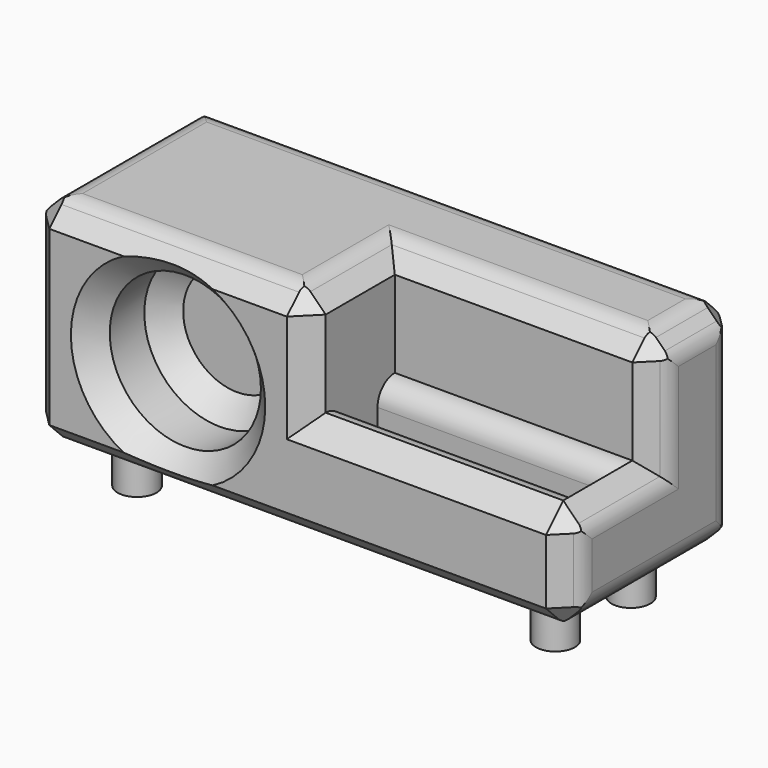
from build123d import *

# Parameters (mm, degrees)
F0_W         = 125
F0_H         = 50
F1_DEPTH     = 50
F2_W         = 60
F2_H         = 25
F3_DEPTH     = 25
F4_R         = 17.5
F5_DEPTH     = 20
F6_T3_DEPTH  = 6.3508529611
F6_T5_DEPTH  = 6.3508529611
F6_T7_DEPTH  = 6.3508529611
F6_T9_DEPTH  = 6.3508529611
F6_T11_DEPTH = 6.3508529611
F6_T13_DEPTH = 6.3508529611
F6_T15_DEPTH = 6.3508529611
F6_T17_DEPTH = 6.3508529611
F6_T19_DEPTH = 6.3508529611
F6_T21_DEPTH = 90.7168298797
F6_T23_DEPTH = 37.8584149398
F6_T25_DEPTH = 72.8584149398
F6_T27_DEPTH = 50.7168298797
F6_T29_DEPTH = 150.7168298797
F6_T31_DEPTH = 75.7168298797
F6_T33_DEPTH = 75.7168298797
F6_T35_DEPTH = 37.8584149398
F6_T37_DEPTH = 50.7168298797
F6_T45_DEPTH = 37.8584149398
F6_T49_DEPTH = 72.8584149398
F6_T56_DEPTH = 37.8584149398
F6_T60_DEPTH = 72.8584149398
F6_T67_DEPTH = 37.8584149398
F6_T71_DEPTH = 37.8584149398
F7_W         = 55
F7_H         = 10
F8_DEPTH     = 10
F9_T1_DEPTH  = 50.3553390594
F9_T3_DEPTH  = 125.3553390595
F9_T5_DEPTH  = 25.3553390594
F9_T7_DEPTH  = 65.3553390594
F9_T9_DEPTH  = 50.3553390593
F9_T11_DEPTH = 25.3553390595
F9_T16_DEPTH = 70.3553390595
F9_T21_DEPTH = 35.3553390594
F9_T26_DEPTH = 35.3553390594
F9_T31_DEPTH = 35.3553390595
F9_T37_DEPTH = 70.3553390595
F9_T41_DEPTH = 35.3553390594
F9_T48_DEPTH = 35.3553390594
F9_T52_DEPTH = 35.3553390595
F10_R        = 4.99999
F11_R        = 4.5
F12_DEPTH    = 10.1


# Not quite as in the source:
# - a fillet or chamfer that OpenCascade refuses, or shapes differently, is made with other operations: its cross-section is extruded or revolved along the edge and cut away or added
# - a fillet or chamfer is up to 0.001 mm smaller than in the source, because OpenCascade refuses the exact size


with BuildPart() as f1:
    # F0 (on Front) → F1 (new body)
    with BuildSketch(Plane.XZ):
        with Locations((4.2377149548, 2.7714315802)):
            Rectangle(F0_W, F0_H)
    extrude(amount=F1_DEPTH)

    # F2 (on face) → F3 (cut)
    with BuildSketch(Plane.XZ.offset(50)):
        with Locations((36.7377149548, 15.2714315802)):
            Rectangle(F2_W, F2_H)
    extrude(amount=-F3_DEPTH, mode=Mode.SUBTRACT)

    # F4 (on face) → F5 (cut)
    with BuildSketch(Plane.XZ.offset(50)):
        with Locations((-25.7622850452, 2.7714315802)):
            Circle(F4_R)
    extrude(amount=-F5_DEPTH, mode=Mode.SUBTRACT)

    # F6: chamfer of 5 on 20 edges, made by hand

    # F6_s1 → F6_t2 (revolve)
    with BuildSketch(Plane.XY.offset(2.7714315802)):
        Polygon((-8.2622850452, -35), (-13.2622850452, -30), (-8.2622850452, -30), align=None)
    revolve(axis=Axis((-25.7622850452, -30, 2.7714315802), (0, -1, 0)))

    # F6_s4 → F6_t3 (cut)
    with BuildSketch(Plane(origin=(24.8363821783, -24.8363821783, 24.8363821783), x_dir=(0.7071067812, 0.7071067812, 0), z_dir=(0.5773502692, -0.5773502692, 0.5773502692))):
        Polygon((-30.5910551251, 3.5946867022), (-34.126589031, -2.5290376548), (-27.0555212191, -2.5290376548), align=None)
    extrude(amount=F6_T3_DEPTH, mode=Mode.SUBTRACT)

    # F6_s6 → F6_t5 (cut)
    with BuildSketch(Plane(origin=(-42.0112388751, -42.0112388751, 42.0112388751), x_dir=(0.7071067812, -0.7071067812, 0), z_dir=(-0.5773502692, -0.5773502692, 0.5773502692))):
        Polygon((-5.8423177835, -17.4401309541), (-9.3778516895, -23.563855311), (-2.3067838776, -23.563855311), align=None)
    extrude(amount=F6_T5_DEPTH, mode=Mode.SUBTRACT)

    # F6_s8 → F6_t7 (cut)
    with BuildSketch(Plane(origin=(36.503048845, -36.503048845, 36.503048845), x_dir=(0.7071067812, 0.7071067812, 0), z_dir=(0.5773502692, -0.5773502692, 0.5773502692))):
        Polygon((29.5130212758, -10.694003464), (25.9774873699, -16.817727821), (33.0485551817, -16.817727821), align=None)
        Polygon((11.8353517461, -41.3126252488), (8.2998178402, -47.4363496058), (15.3708856521, -47.4363496058), align=None)
    extrude(amount=F6_T7_DEPTH, mode=Mode.SUBTRACT)

    # F6_s10 → F6_t9 (cut)
    with BuildSketch(Plane(origin=(28.1697155117, 28.1697155117, 28.1697155117), x_dir=(-0.7071067812, 0.7071067812, 0), z_dir=(0.5773502692, 0.5773502692, 0.5773502692))):
        Polygon((-47.1906908055, -0.4877962024), (-43.6551568995, -6.6115205594), (-50.7262247114, -6.6115205594), align=None)
    extrude(amount=F6_T9_DEPTH, mode=Mode.SUBTRACT)

    # F6_s12 → F6_t11 (cut)
    with BuildSketch(Plane(origin=(-25.3445722085, 25.3445722085, 25.3445722085), x_dir=(-0.7071067812, -0.7071067812, 0), z_dir=(-0.5773502692, 0.5773502692, 0.5773502692))):
        Polygon((41.1976568429, 2.9722835691), (37.6621229369, -3.1514407878), (44.7331907488, -3.1514407878), align=None)
    extrude(amount=F6_T11_DEPTH, mode=Mode.SUBTRACT)

    # F6_s14 → F6_t13 (cut)
    with BuildSketch(Plane(origin=(-40.1636178217, -40.1636178217, -40.1636178217), x_dir=(0.7071067812, -0.7071067812, 0), z_dir=(-0.5773502692, -0.5773502692, -0.5773502692))):
        Polygon((-9.3778516895, 28.08958413), (-2.3067838776, 28.08958413), (-5.8423177835, 21.9658597731), align=None)
    extrude(amount=F6_T13_DEPTH, mode=Mode.SUBTRACT)

    # F6_s16 → F6_t15 (cut)
    with BuildSketch(Plane(origin=(26.3220944582, 26.3220944582, -26.3220944582), x_dir=(-0.7071067812, 0.7071067812, 0), z_dir=(0.5773502692, 0.5773502692, -0.5773502692))):
        Polygon((-43.6551568995, 11.1372493784), (-50.7262247114, 11.1372493784), (-47.1906908055, 5.0135250214), align=None)
    extrude(amount=F6_T15_DEPTH, mode=Mode.SUBTRACT)

    # F6_s18 → F6_t17 (cut)
    with BuildSketch(Plane(origin=(42.9887611249, -42.9887611249, -42.9887611249), x_dir=(0.7071067812, 0.7071067812, 0), z_dir=(0.5773502692, -0.5773502692, -0.5773502692))):
        Polygon((8.2998178402, 31.5496639016), (15.3708856521, 31.5496639016), (11.8353517461, 25.4259395446), align=None)
    extrude(amount=F6_T17_DEPTH, mode=Mode.SUBTRACT)

    # F6_s20 → F6_t19 (cut)
    with BuildSketch(Plane(origin=(-23.496951155, 23.496951155, -23.496951155), x_dir=(-0.7071067812, -0.7071067812, 0), z_dir=(-0.5773502692, 0.5773502692, -0.5773502692))):
        Polygon((37.6621229369, 7.6771696068), (44.7331907488, 7.6771696068), (41.1976568429, 1.5534452499), align=None)
    extrude(amount=F6_T19_DEPTH, mode=Mode.SUBTRACT)

    # F6_s22 → F6_t21 (cut)
    with BuildSketch(Plane.YZ.offset(-71.120699985)):
        Polygon((-45, 27.7714315802), (-50, 22.7714315802), (-50, 27.7714315802), align=None)
    extrude(amount=F6_T21_DEPTH, mode=Mode.SUBTRACT)

    # F6_s24 → F6_t23 (cut)
    with BuildSketch(Plane.XZ.offset(25)):
        Polygon((1.7377149548, 27.7714315802), (6.7377149548, 22.7714315802), (6.7377149548, 27.7714315802), align=None)
        Polygon((66.7377149548, -2.2285684198), (61.7377149548, 2.7714315802), (66.7377149548, 2.7714315802), align=None)
    extrude(amount=F6_T23_DEPTH, mode=Mode.SUBTRACT)

    # F6_s26 → F6_t25 (cut)
    with BuildSketch(Plane.YZ.offset(6.7377149548)):
        Polygon((-20, 27.7714315802), (-25, 22.7714315802), (-25, 27.7714315802), align=None)
        Polygon((-50, -2.2285684198), (-45, 2.7714315802), (-50, 2.7714315802), align=None)
    extrude(amount=F6_T25_DEPTH, mode=Mode.SUBTRACT)

    # F6_s28 → F6_t27 (cut)
    with BuildSketch(Plane.XZ.offset(-12.8584149398)):
        Polygon((61.7377149548, 27.7714315802), (66.7377149548, 22.7714315802), (66.7377149548, 27.7714315802), align=None)
    extrude(amount=F6_T27_DEPTH, mode=Mode.SUBTRACT)

    # F6_s30 → F6_t29 (cut)
    with BuildSketch(Plane.YZ.offset(-71.120699985)):
        Polygon((-5, 27.7714315802), (0, 22.7714315802), (0, 27.7714315802), align=None)
        Polygon((-50, -17.2285684198), (-45, -22.2285684198), (-50, -22.2285684198), align=None)
        Polygon((0, -17.2285684198), (-5, -22.2285684198), (0, -22.2285684198), align=None)
    extrude(amount=F6_T29_DEPTH, mode=Mode.SUBTRACT)

    # F6_s32 → F6_t31 (cut)
    with BuildSketch(Plane.XZ.offset(-12.8584149398)):
        Polygon((-53.2622850452, 27.7714315802), (-58.2622850452, 22.7714315802), (-58.2622850452, 27.7714315802), align=None)
        Polygon((66.7377149548, -17.2285684198), (61.7377149548, -22.2285684198), (66.7377149548, -22.2285684198), align=None)
        Polygon((-58.2622850452, -17.2285684198), (-53.2622850452, -22.2285684198), (-58.2622850452, -22.2285684198), align=None)
    extrude(amount=F6_T31_DEPTH, mode=Mode.SUBTRACT)

    # F6_s34 → F6_t33 (cut)
    with BuildSketch(Plane.XY.offset(-35.0869833596)):
        Polygon((-58.2622850452, -45), (-53.2622850452, -50), (-58.2622850452, -50), align=None)
        Polygon((61.7377149548, 0), (66.7377149548, -5), (66.7377149548, 0), align=None)
        Polygon((-53.2622850452, 0), (-58.2622850452, -5), (-58.2622850452, 0), align=None)
    extrude(amount=F6_T33_DEPTH, mode=Mode.SUBTRACT)

    # F6_s36 → F6_t35 (cut)
    with BuildSketch(Plane.XY.offset(2.7714315802)):
        Polygon((1.7377149548, -50), (6.7377149548, -45), (6.7377149548, -50), align=None)
        Polygon((61.7377149548, -25), (66.7377149548, -20), (66.7377149548, -25), align=None)
    extrude(amount=F6_T35_DEPTH, mode=Mode.SUBTRACT)

    # F6_s38 → F6_t37 (cut)
    with BuildSketch(Plane.XY.offset(-35.0869833596)):
        Polygon((61.7377149548, -50), (66.7377149548, -45), (66.7377149548, -50), align=None)
    extrude(amount=F6_T37_DEPTH, mode=Mode.SUBTRACT)

    # F6_s39 → F6_t40 (revolve, cut)
    with BuildSketch(Plane.XY.offset(2.7714315802)):
        Polygon((-3.2622850452, -50), (-8.2622850452, -45), (-8.2622850452, -50), align=None)
    revolve(axis=Axis((-25.7622850452, -50, 2.7714315802), (0, -1, 0)), mode=Mode.SUBTRACT)


with BuildPart() as f6_tool43:
    # F6_s44 → F6_t45 (new body)
    with BuildSketch(Plane.XZ.offset(50)):
        Polygon((1.7377149548, 27.7714315802), (6.7377149548, 22.7714315802), (6.7377149548, 27.7714315802), align=None)
    extrude(amount=-F6_T45_DEPTH)

    split(bisect_by=Plane.XZ.offset(25), keep=Keep.BOTTOM)


with BuildPart() as f6_tool47:
    # F6_s48 → F6_t49 (new body)
    with BuildSketch(Plane.YZ.offset(66.7377149548)):
        Polygon((-20, 27.7714315802), (-25, 22.7714315802), (-25, 27.7714315802), align=None)
    extrude(amount=-F6_T49_DEPTH)

    split(bisect_by=Plane.YZ.offset(6.7377149548), keep=Keep.BOTTOM)


with BuildPart() as f6_tool43_1:
    add(f6_tool43.part)

    # F6_t51: intersect F6_tool47
    add(f6_tool47.part, mode=Mode.INTERSECT)


with BuildPart() as f1_1:
    add(f1.part)

    # F6_t41: cut F6_tool43
    add(f6_tool43_1.part, mode=Mode.SUBTRACT)


with BuildPart() as f6_tool54:
    # F6_s55 → F6_t56 (new body)
    with BuildSketch(Plane.XY.offset(27.7714315802)):
        Polygon((1.7377149548, -50), (6.7377149548, -45), (6.7377149548, -50), align=None)
    extrude(amount=-F6_T56_DEPTH)

    split(bisect_by=Plane.XY.offset(2.7714315802), keep=Keep.BOTTOM)


with BuildPart() as f6_tool58:
    # F6_s59 → F6_t60 (new body)
    with BuildSketch(Plane.YZ.offset(-6.120699985)):
        Polygon((-50, -2.2285684198), (-45, 2.7714315802), (-50, 2.7714315802), align=None)
    extrude(amount=F6_T60_DEPTH)

    split(bisect_by=Plane.YZ.offset(6.7377149548), keep=Keep.BOTTOM)


with BuildPart() as f6_tool54_1:
    add(f6_tool54.part)

    # F6_t62: intersect F6_tool58
    add(f6_tool58.part, mode=Mode.INTERSECT)


with BuildPart() as f1_2:
    add(f1_1.part)

    # F6_t52: cut F6_tool54
    add(f6_tool54_1.part, mode=Mode.SUBTRACT)


with BuildPart() as f6_tool65:
    # F6_s66 → F6_t67 (new body)
    with BuildSketch(Plane.XY.offset(-10.0869833596)):
        Polygon((61.7377149548, -25), (66.7377149548, -20), (66.7377149548, -25), align=None)
    extrude(amount=F6_T67_DEPTH)

    split(bisect_by=Plane.XY.offset(2.7714315802), keep=Keep.BOTTOM)


with BuildPart() as f6_tool69:
    # F6_s70 → F6_t71 (new body)
    with BuildSketch(Plane.XZ.offset(50)):
        Polygon((66.7377149548, -2.2285684198), (61.7377149548, 2.7714315802), (66.7377149548, 2.7714315802), align=None)
    extrude(amount=-F6_T71_DEPTH)

    split(bisect_by=Plane.XZ.offset(25), keep=Keep.BOTTOM)


with BuildPart() as f6_tool65_1:
    add(f6_tool65.part)

    # F6_t73: intersect F6_tool69
    add(f6_tool69.part, mode=Mode.INTERSECT)


with BuildPart() as f1_3:
    add(f1_2.part)

    # F6_t63: cut F6_tool65
    add(f6_tool65_1.part, mode=Mode.SUBTRACT)

    # F7 (on face) → F8 (cut)
    with BuildSketch(Plane.XY.offset(2.7714315802)):
        with Locations((34.2377149548, -35)):
            Rectangle(F7_W, F7_H)
    extrude(amount=-F8_DEPTH, mode=Mode.SUBTRACT)

    # F9: fillet of radius 5 on 24 edges, made by hand

    # F9_s2 → F9_t1 (cut)
    with BuildSketch(Plane.XZ.offset(-0.1776695297)):
        with BuildLine():
            ThreePointArc((-51.1912172333, 27.7714315802), (-53.1046343952, 27.3908292427), (-54.7267511393, 26.3069654861))
            Line((-54.7267511393, 26.3069654861), (-53.2622850452, 27.7714315802))
            Line((-53.2622850452, 27.7714315802), (-51.1912172333, 27.7714315802))
        make_face()
        with BuildLine():
            ThreePointArc((63.2021810489, -20.7641023257), (61.5800643047, -21.8479660824), (59.6666471429, -22.2285684198))
            Line((59.6666471429, -22.2285684198), (61.7377149548, -22.2285684198))
            Line((61.7377149548, -22.2285684198), (63.2021810489, -20.7641023257))
        make_face()
        with BuildLine():
            ThreePointArc((-54.7267511393, -20.7641023257), (-53.1046343951, -21.8479660824), (-51.1912172333, -22.2285684198))
            Line((-51.1912172333, -22.2285684198), (-53.2622850452, -22.2285684198))
            Line((-53.2622850452, -22.2285684198), (-54.7267511393, -20.7641023257))
        make_face()
        with BuildLine():
            ThreePointArc((66.7377149548, -15.1575006079), (66.3571126174, -17.0709177697), (65.2732488608, -18.6930345138))
            Line((65.2732488608, -18.6930345138), (66.7377149548, -17.2285684198))
            Line((66.7377149548, -17.2285684198), (66.7377149548, -15.1575006079))
        make_face()
        with BuildLine():
            ThreePointArc((-58.2622850452, -15.157500608), (-57.8816827077, -17.0709177698), (-56.7978189511, -18.6930345139))
            Line((-56.7978189511, -18.6930345139), (-58.2622850452, -17.2285684198))
            Line((-58.2622850452, -17.2285684198), (-58.2622850452, -15.157500608))
        make_face()
        with BuildLine():
            ThreePointArc((-56.7978189511, 24.2358976743), (-57.8816827077, 22.6137809302), (-58.2622850452, 20.7003637684))
            Line((-58.2622850452, 20.7003637684), (-58.2622850452, 22.7714315802))
            Line((-58.2622850452, 22.7714315802), (-56.7978189511, 24.2358976743))
        make_face()
    extrude(amount=F9_T1_DEPTH, mode=Mode.SUBTRACT)

    # F9_s4 → F9_t3 (cut)
    with BuildSketch(Plane.YZ.offset(-58.4399545749)):
        with BuildLine():
            ThreePointArc((-7.0710678119, 27.7714315802), (-5.15765065, 27.3908292427), (-3.5355339059, 26.3069654861))
            Line((-3.5355339059, 26.3069654861), (-5, 27.7714315802))
            Line((-5, 27.7714315802), (-7.0710678119, 27.7714315802))
        make_face()
        with BuildLine():
            ThreePointArc((-3.5355339059, -20.7641023257), (-5.1576506501, -21.8479660824), (-7.0710678119, -22.2285684198))
            Line((-7.0710678119, -22.2285684198), (-5, -22.2285684198))
            Line((-5, -22.2285684198), (-3.5355339059, -20.7641023257))
        make_face()
        with BuildLine():
            ThreePointArc((-46.4644660941, -20.7641023257), (-44.8423493499, -21.8479660824), (-42.9289321881, -22.2285684198))
            Line((-42.9289321881, -22.2285684198), (-45, -22.2285684198))
            Line((-45, -22.2285684198), (-46.4644660941, -20.7641023257))
        make_face()
        with BuildLine():
            ThreePointArc((0, -15.1575006079), (-0.3806023374, -17.0709177698), (-1.4644660941, -18.6930345139))
            Line((-1.4644660941, -18.6930345139), (0, -17.2285684198))
            Line((0, -17.2285684198), (0, -15.1575006079))
        make_face()
        with BuildLine():
            ThreePointArc((-1.4644660941, 24.2358976743), (-0.3806023374, 22.6137809302), (0, 20.7003637683))
            Line((0, 20.7003637683), (0, 22.7714315802))
            Line((0, 22.7714315802), (-1.4644660941, 24.2358976743))
        make_face()
    extrude(amount=F9_T3_DEPTH, mode=Mode.SUBTRACT)

    # F9_s6 → F9_t5 (cut)
    with BuildSketch(Plane.XZ.offset(-0.1776695297)):
        with BuildLine():
            ThreePointArc((59.6666471429, 27.7714315802), (61.5800643048, 27.3908292427), (63.2021810489, 26.3069654861))
            Line((63.2021810489, 26.3069654861), (61.7377149548, 27.7714315802))
            Line((61.7377149548, 27.7714315802), (59.6666471429, 27.7714315802))
        make_face()
        with BuildLine():
            ThreePointArc((65.2732488608, 24.2358976742), (66.3571126174, 22.6137809301), (66.7377149548, 20.7003637683))
            Line((66.7377149548, 20.7003637683), (66.7377149548, 22.7714315802))
            Line((66.7377149548, 22.7714315802), (65.2732488608, 24.2358976742))
        make_face()
    extrude(amount=F9_T5_DEPTH, mode=Mode.SUBTRACT)

    # F9_s8 → F9_t7 (cut)
    with BuildSketch(Plane.YZ.offset(-58.4399545749)):
        with BuildLine():
            ThreePointArc((-42.9289321881, 27.7714315802), (-44.84234935, 27.3908292427), (-46.4644660941, 26.3069654861))
            Line((-46.4644660941, 26.3069654861), (-45, 27.7714315802))
            Line((-45, 27.7714315802), (-42.9289321881, 27.7714315802))
        make_face()
    extrude(amount=F9_T7_DEPTH, mode=Mode.SUBTRACT)

    # F9_s10 → F9_t9 (cut)
    with BuildSketch(Plane.XY.offset(-22.4062379495)):
        with BuildLine():
            ThreePointArc((59.6666471429, 0), (61.5800643048, -0.3806023374), (63.2021810489, -1.4644660941))
            Line((63.2021810489, -1.4644660941), (61.7377149548, 0))
            Line((61.7377149548, 0), (59.6666471429, 0))
        make_face()
        with BuildLine():
            ThreePointArc((-51.1912172333, 0), (-53.1046343952, -0.3806023374), (-54.7267511393, -1.4644660941))
            Line((-54.7267511393, -1.4644660941), (-53.2622850452, 0))
            Line((-53.2622850452, 0), (-51.1912172333, 0))
        make_face()
        with BuildLine():
            ThreePointArc((66.7377149548, -7.0710678119), (66.3571126174, -5.1576506501), (65.2732488608, -3.535533906))
            Line((65.2732488608, -3.535533906), (66.7377149548, -5))
            Line((66.7377149548, -5), (66.7377149548, -7.0710678119))
        make_face()
        with BuildLine():
            ThreePointArc((-58.2622850452, -7.0710678118), (-57.8816827077, -5.15765065), (-56.7978189511, -3.5355339059))
            Line((-56.7978189511, -3.5355339059), (-58.2622850452, -5))
            Line((-58.2622850452, -5), (-58.2622850452, -7.0710678118))
        make_face()
        with BuildLine():
            ThreePointArc((-58.2622850452, -42.9289321882), (-57.8816827077, -44.84234935), (-56.7978189511, -46.4644660941))
            Line((-56.7978189511, -46.4644660941), (-58.2622850452, -45))
            Line((-58.2622850452, -45), (-58.2622850452, -42.9289321882))
        make_face()
    extrude(amount=F9_T9_DEPTH, mode=Mode.SUBTRACT)

    # F9_s12 → F9_t11 (cut)
    with BuildSketch(Plane.XY.offset(-22.4062379496)):
        with BuildLine():
            ThreePointArc((66.7377149548, -42.9289321881), (66.3571126174, -44.8423493499), (65.2732488608, -46.464466094))
            Line((65.2732488608, -46.464466094), (66.7377149548, -45))
            Line((66.7377149548, -45), (66.7377149548, -42.9289321881))
        make_face()
    extrude(amount=F9_T11_DEPTH, mode=Mode.SUBTRACT)


with BuildPart() as f9_tool14:
    # F9_s15 → F9_t16 (new body)
    with BuildSketch(Plane.YZ.offset(-3.439954575)):
        with BuildLine():
            ThreePointArc((-17.9289321882, 27.7714315802), (-19.84234935, 27.3908292427), (-21.4644660941, 26.3069654861))
            Line((-21.4644660941, 26.3069654861), (-20, 27.7714315802))
            Line((-20, 27.7714315802), (-17.9289321882, 27.7714315802))
        make_face()
    extrude(amount=F9_T16_DEPTH)

    split(bisect_by=Plane(origin=(14.7545732675, 0, 14.7545732675), x_dir=(0, 1, 0), z_dir=(0.7071067812, 0, 0.7071067812)), keep=Keep.TOP)


with BuildPart() as f1_4:
    add(f1_3.part)

    # F9_t13: cut F9_tool14
    add(f9_tool14.part, mode=Mode.SUBTRACT)


with BuildPart() as f9_tool19:
    # F9_s20 → F9_t21 (new body)
    with BuildSketch(Plane.XZ.offset(50.1776695297)):
        with BuildLine():
            ThreePointArc((-0.333352857, 27.7714315802), (1.5800643048, 27.3908292427), (3.2021810489, 26.3069654861))
            Line((3.2021810489, 26.3069654861), (1.7377149548, 27.7714315802))
            Line((1.7377149548, 27.7714315802), (-0.333352857, 27.7714315802))
        make_face()
    extrude(amount=-F9_T21_DEPTH)

    split(bisect_by=Plane(origin=(0, -23.8857157901, 23.8857157901), x_dir=(1, 0, 0), z_dir=(0, -0.7071067812, 0.7071067812)), keep=Keep.TOP)


with BuildPart() as f1_5:
    add(f1_4.part)

    # F9_t18: cut F9_tool19
    add(f9_tool19.part, mode=Mode.SUBTRACT)


with BuildPart() as f9_tool24:
    # F9_s25 → F9_t26 (new body)
    with BuildSketch(Plane.XZ.offset(14.8223304703)):
        with BuildLine():
            ThreePointArc((66.7377149548, -4.2996362317), (66.3571126173, -2.3862190699), (65.2732488607, -0.7641023257))
            Line((65.2732488607, -0.7641023257), (66.7377149548, -2.2285684198))
            Line((66.7377149548, -2.2285684198), (66.7377149548, -4.2996362317))
        make_face()
    extrude(amount=F9_T26_DEPTH)

    split(bisect_by=Plane(origin=(43.3688574774, -43.3688574774, 0), x_dir=(0, 0, 1), z_dir=(0.7071067812, -0.7071067812, 0)), keep=Keep.TOP)


with BuildPart() as f1_6:
    add(f1_5.part)

    # F9_t23: cut F9_tool24
    add(f9_tool24.part, mode=Mode.SUBTRACT)


with BuildPart() as f9_tool29:
    # F9_s30 → F9_t31 (new body)
    with BuildSketch(Plane.XY.offset(27.94910111)):
        with BuildLine():
            ThreePointArc((66.7377149548, -17.9289321881), (66.3571126174, -19.8423493499), (65.2732488608, -21.464466094))
            Line((65.2732488608, -21.464466094), (66.7377149548, -20))
            Line((66.7377149548, -20), (66.7377149548, -17.9289321881))
        make_face()
    extrude(amount=-F9_T31_DEPTH)

    split(bisect_by=Plane(origin=(32.2545732675, 0, 32.2545732675), x_dir=(0, 1, 0), z_dir=(0.7071067812, 0, 0.7071067812)), keep=Keep.TOP)


with BuildPart() as f1_7:
    add(f1_6.part)

    # F9_t28: cut F9_tool29
    add(f9_tool29.part, mode=Mode.SUBTRACT)


with BuildPart() as f9_tool35:
    # F9_s36 → F9_t37 (new body)
    with BuildSketch(Plane.YZ.offset(-3.439954575)):
        with BuildLine():
            ThreePointArc((-17.9289321882, 27.7714315802), (-19.84234935, 27.3908292427), (-21.4644660941, 26.3069654861))
            Line((-21.4644660941, 26.3069654861), (-20, 27.7714315802))
            Line((-20, 27.7714315802), (-17.9289321882, 27.7714315802))
        make_face()
    extrude(amount=F9_T37_DEPTH)

    split(bisect_by=Plane(origin=(14.7545732675, 0, 14.7545732675), x_dir=(0, 1, 0), z_dir=(-0.7071067812, 0, -0.7071067812)), keep=Keep.TOP)


with BuildPart() as f9_tool39:
    # F9_s40 → F9_t41 (new body)
    with BuildSketch(Plane.XZ.offset(50.1776695297)):
        with BuildLine():
            ThreePointArc((-0.333352857, 27.7714315802), (1.5800643048, 27.3908292427), (3.2021810489, 26.3069654861))
            Line((3.2021810489, 26.3069654861), (1.7377149548, 27.7714315802))
            Line((1.7377149548, 27.7714315802), (-0.333352857, 27.7714315802))
        make_face()
    extrude(amount=-F9_T41_DEPTH)

    split(bisect_by=Plane(origin=(0, -23.8857157901, 23.8857157901), x_dir=(1, 0, 0), z_dir=(0, 0.7071067812, -0.7071067812)), keep=Keep.TOP)


with BuildPart() as f9_tool35_1:
    add(f9_tool35.part)

    # F9_t43: intersect F9_tool39
    add(f9_tool39.part, mode=Mode.INTERSECT)


with BuildPart() as f1_8:
    add(f1_7.part)

    # F9_t33: cut F9_tool35
    add(f9_tool35_1.part, mode=Mode.SUBTRACT)


with BuildPart() as f9_tool46:
    # F9_s47 → F9_t48 (new body)
    with BuildSketch(Plane.XZ.offset(14.8223304703)):
        with BuildLine():
            ThreePointArc((66.7377149548, -4.2996362317), (66.3571126173, -2.3862190699), (65.2732488607, -0.7641023257))
            Line((65.2732488607, -0.7641023257), (66.7377149548, -2.2285684198))
            Line((66.7377149548, -2.2285684198), (66.7377149548, -4.2996362317))
        make_face()
    extrude(amount=F9_T48_DEPTH)

    split(bisect_by=Plane(origin=(43.3688574774, -43.3688574774, 0), x_dir=(0, 0, 1), z_dir=(-0.7071067812, 0.7071067812, 0)), keep=Keep.TOP)


with BuildPart() as f9_tool50:
    # F9_s51 → F9_t52 (new body)
    with BuildSketch(Plane.XY.offset(27.94910111)):
        with BuildLine():
            ThreePointArc((66.7377149548, -17.9289321881), (66.3571126174, -19.8423493499), (65.2732488608, -21.464466094))
            Line((65.2732488608, -21.464466094), (66.7377149548, -20))
            Line((66.7377149548, -20), (66.7377149548, -17.9289321881))
        make_face()
    extrude(amount=-F9_T52_DEPTH)

    split(bisect_by=Plane(origin=(32.2545732675, 0, 32.2545732675), x_dir=(0, 1, 0), z_dir=(-0.7071067812, 0, -0.7071067812)), keep=Keep.TOP)


with BuildPart() as f9_tool46_1:
    add(f9_tool46.part)

    # F9_t54: intersect F9_tool50
    add(f9_tool50.part, mode=Mode.INTERSECT)


with BuildPart() as f1_9:
    add(f1_8.part)

    # F9_t44: cut F9_tool46
    add(f9_tool46_1.part, mode=Mode.SUBTRACT)

    # F10 (radius 5 in the source; OpenCascade refuses exactly that, so slightly less here)
    f10_edges = [f1_9.edges().sort_by_distance(p)[0] for p in [
        (34.237715, -30, 2.771432),
        (34.237715, -40, 2.771432),
    ]]
    fillet(f10_edges, radius=F10_R)

    # F11 (on face) → F12 (join)
    with BuildSketch(Plane(origin=(0, 0, -22.2285684198), x_dir=(1, 0, 0), z_dir=(0, 0, -1))):
        with Locations((-44.1912172333, 35.9289321881)):
            Circle(F11_R)
        with Locations((-44.1912172333, 14.0710678119)):
            Circle(F11_R)
        with Locations((52.666647143, 14.0710678119)):
            Circle(F11_R)
        with Locations((52.666647143, 35.9289321881)):
            Circle(F11_R)
    extrude(amount=F12_DEPTH)


solid = f1_9.part
